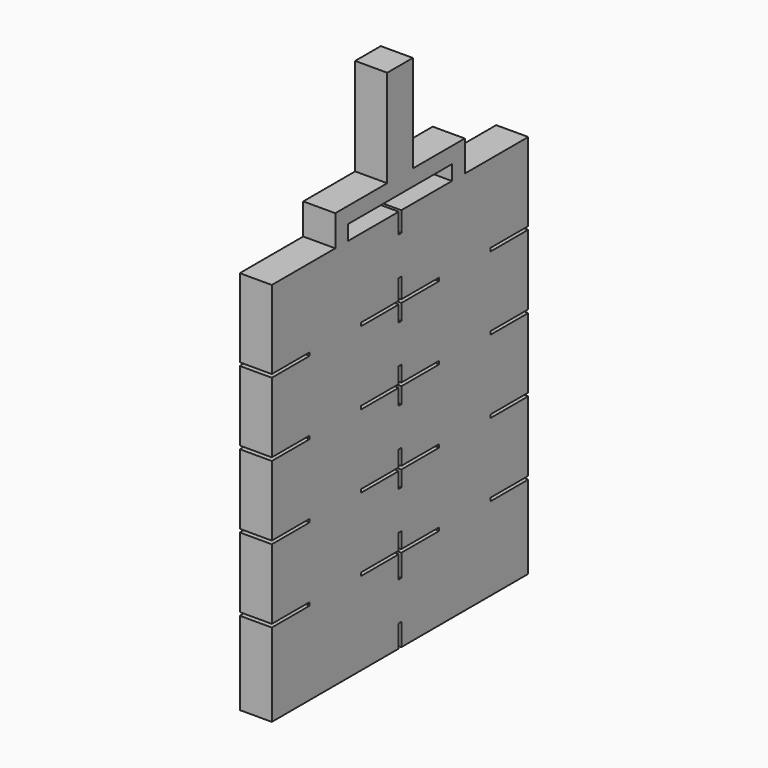
from build123d import *

# Parameters (mm, degrees)
F1_DEPTH = 5


# Not quite as in the source:
# - a feature names something its author has since deleted; it is built from what else it names


with BuildPart() as f1:
    # F0 (on Right) → F1 (new body)
    with BuildSketch(Plane.YZ):
        Polygon((12.375, 0), (0, 0), (0, -12.238), (7.3750000447, -12.238), (7.3750000447, -12.738), (0, -12.738), (0, -23.672), (7.3750000447, -23.672), (7.3750000447, -24.172), (0, -24.172), (0, -35.106), (7.3750000447, -35.106), (7.3750000447, -35.606), (0, -35.606), (0, -46.54), (7.3750000447, -46.54), (7.3750000447, -47.04), (0, -47.04), (0, -60), (24.75, -60), (24.75, -56.52), (25.25, -56.52), (25.25, -60), (50, -60), (50, -47.04), (42.6249988377, -47.04), (42.6249988377, -46.54), (50, -46.54), (50, -35.606), (42.6249988377, -35.606), (42.6249988377, -35.106), (50, -35.106), (50, -24.172), (42.6249988377, -24.172), (42.6249988377, -23.672), (50, -23.672), (50, -12.738), (42.6249988377, -12.738), (42.6249988377, -12.238), (50, -12.238), (50, 0), (37.625, 0), (37.625, 4.8238829523), (27.5, 4.8238829523), (27.5, 9.8238829523), (27.5, 20), (22.5, 20), (22.5, 9.8238829523), (22.5, 4.8238829523), (12.375, 4.8238829523), align=None)
        Polygon((25.25, -44.073), (25.25, -46.54), (32.625, -46.54), (32.625, -47.04), (25.25, -47.04), (25.25, -50.52), (24.75, -50.52), (24.75, -47.04), (17.375, -47.04), (17.375, -46.54), (24.75, -46.54), (24.75, -44.073), align=None, mode=Mode.SUBTRACT)
        Polygon((25.25, -32.639), (25.25, -35.106), (32.625, -35.106), (32.625, -35.606), (25.25, -35.606), (25.25, -38.073), (24.75, -38.073), (24.75, -35.606), (17.375, -35.606), (17.375, -35.106), (24.75, -35.106), (24.75, -32.639), align=None, mode=Mode.SUBTRACT)
        Polygon((25.25, -21.205), (25.25, -23.672), (32.625, -23.672), (32.625, -24.172), (25.25, -24.172), (25.25, -26.639), (24.75, -26.639), (24.75, -24.172), (17.375, -24.172), (17.375, -23.672), (24.75, -23.672), (24.75, -21.205), align=None, mode=Mode.SUBTRACT)
        Polygon((25.25, -9.119), (25.25, -12.238), (32.625, -12.238), (32.625, -12.738), (25.25, -12.738), (25.25, -15.205), (24.75, -15.205), (24.75, -12.738), (17.375, -12.738), (17.375, -12.238), (24.75, -12.238), (24.75, -9.119), align=None, mode=Mode.SUBTRACT)
        Polygon((25.25, -1.304), (25.25, -3.119), (24.75, -3.119), (24.75, 0), (14.875, 0), (14.875, 2.3238829523), (35.125, 2.3238829523), (35.125, 0), (25.25, 0), align=None, mode=Mode.SUBTRACT)
    extrude(amount=F1_DEPTH)


solid = f1.part
